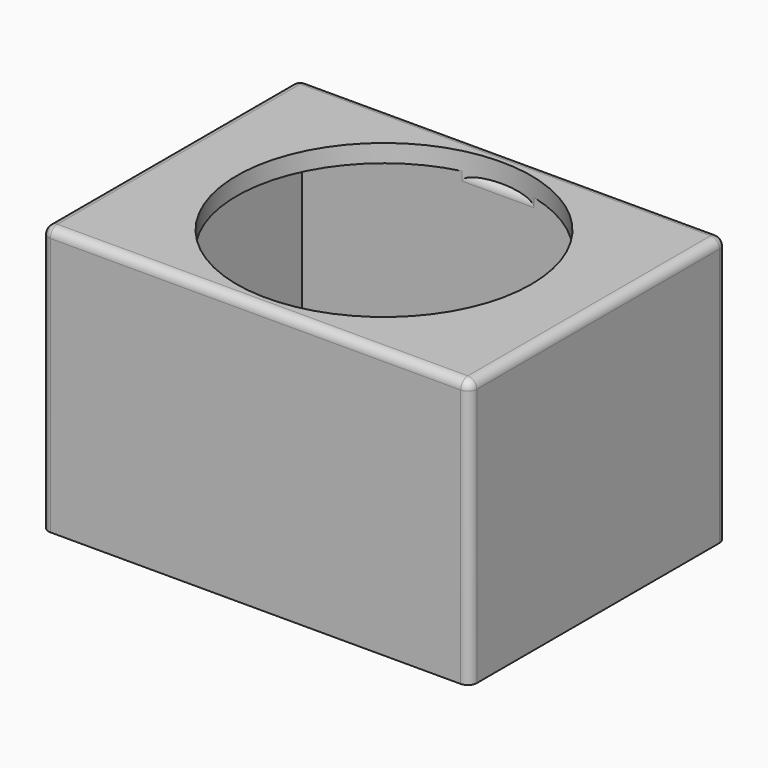
from build123d import *

# Parameters (mm, degrees)
F0_W         = 609.6
F0_H         = 457.2
F1_DEPTH     = 381
F2_R         = 12.7
F3_T         = -25.4
F4_R         = 209.55
F5_DEPTH     = 25.4
F6_T4_DEPTH  = 165.8906734034
F6_S5_R      = 209.55
F6_T6_DEPTH  = 85
F6_T10_DEPTH = 165.8906734034
F6_S11_R     = 209.55
F6_T12_DEPTH = 85


# Not quite as in the source:
# - a fillet or chamfer that OpenCascade refuses, or shapes differently, is made with other operations: its cross-section is extruded or revolved along the edge and cut away or added


with BuildPart() as f1:
    # F0 (on Top) → F1 (new body)
    with BuildSketch(Plane.XY):
        Rectangle(F0_W, F0_H)
    extrude(amount=F1_DEPTH)

    # F2
    f2_edges = [f1.edges().sort_by_distance(p)[0] for p in [
        (304.8, 0, 381),
        (0, 228.6, 381),
        (-304.8, 0, 381),
        (0, -228.6, 381),
        (-304.8, -228.6, 190.5),
        (304.8, -228.6, 190.5),
        (304.8, 228.6, 190.5),
        (-304.8, 228.6, 190.5),
    ]]
    fillet(f2_edges, radius=F2_R)

    # F3 (hollow: no face is removed)
    offset(amount=F3_T, mode=Mode.SUBTRACT)

    # F4 (on face) → F5 (cut)
    with BuildSketch(Plane.XY.offset(381)):
        Circle(F4_R)
    extrude(amount=-F5_DEPTH, mode=Mode.SUBTRACT)

    # F6: fillet of radius 12.7 on 2 edges, made by hand


with BuildPart() as f6_tool2:
    # F6_s3 → F6_t4 (new body)
    with BuildSketch(Plane.YZ.offset(82.9453367017)):
        with BuildLine():
            ThreePointArc((-215.9, 355.6), (-206.9197438789, 351.8802561211), (-203.2, 342.9))
            Line((-203.2, 342.9), (-203.2, 355.6))
            Line((-203.2, 355.6), (-215.9, 355.6))
        make_face()
    extrude(amount=-F6_T4_DEPTH)

    # F6_s5 → F6_t6 (intersect, symmetric)
    with BuildSketch(Plane.XY.offset(349.3)):
        Circle(F6_S5_R)
    extrude(amount=F6_T6_DEPTH, both=True, mode=Mode.INTERSECT)


with BuildPart() as f1_1:
    add(f1.part)

    # F6_t1: cut F6_tool2
    add(f6_tool2.part, mode=Mode.SUBTRACT)


with BuildPart() as f6_tool8:
    # F6_s9 → F6_t10 (new body)
    with BuildSketch(Plane.YZ.offset(-82.9453367017)):
        with BuildLine():
            ThreePointArc((215.9, 355.6), (206.9197438789, 351.8802561211), (203.2, 342.9))
            Line((203.2, 342.9), (203.2, 355.6))
            Line((203.2, 355.6), (215.9, 355.6))
        make_face()
    extrude(amount=F6_T10_DEPTH)

    # F6_s11 → F6_t12 (intersect, symmetric)
    with BuildSketch(Plane.XY.offset(349.3)):
        Circle(F6_S11_R)
    extrude(amount=F6_T12_DEPTH, both=True, mode=Mode.INTERSECT)


with BuildPart() as f1_2:
    add(f1_1.part)

    # F6_t7: cut F6_tool8
    add(f6_tool8.part, mode=Mode.SUBTRACT)


solid = f1_2.part
